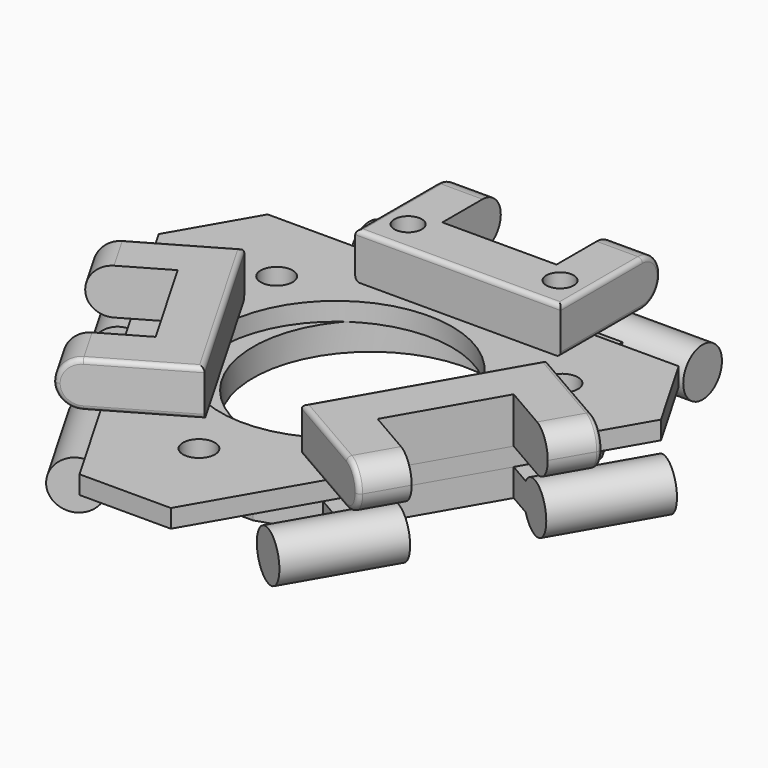
from build123d import *

# Parameters (mm, degrees)
F0_R      = 12.9
F1_DEPTH  = 3
F2_R      = 1.75
F3_DEPTH  = 3.001
F4_R      = 2.65
F5_DEPTH  = 12
F6_R      = 2.65
F7_DEPTH  = 12
F8_R      = 2.65
F9_DEPTH  = 12
F10_R     = 2.65
F11_DEPTH = 12
F12_R     = 2.65
F13_DEPTH = 12
F14_R     = 2.65
F15_DEPTH = 12
F16_R     = 1.75
F16_R_2   = 12.7
F17_DEPTH = 2
F18_SIZE  = 10
F20_DEPTH = 5
F21_R     = 2.49999
F21_2_R   = 2.49999
F21_3_R   = 2.49999
F22_R     = 0.5
F22_2_R   = 0.5
F22_3_R   = 0.5
F23_R     = 1.5
F24_DEPTH = 11.151


# Not quite as in the source:
# - a fillet or chamfer is up to 0.001 mm smaller than in the source, because OpenCascade refuses the exact size


with BuildPart() as f1:
    # F0 (on Top) → F1 (new body)
    with BuildSketch(Plane.XY):
        Polygon((16.0075136901, 22.7174561645), (11.25, 26.956246243), (11.25, 31.956246243), (6.25, 31.956246243), (6.25, 26.956246243), (-6.25, 26.956246243), (-6.25, 31.956246243), (-11.25, 31.956246243), (-11.25, 26.956246243), (-16.0075136901, 22.7174561645), (-19.6075136901, 16.4820732572), (-20.8996567344, 10.2425505034), (-25.2297837534, 7.7425505034), (-22.7297837534, 3.4124234845), (-18.3996567344, 5.9124234845), (-12.1496567344, -4.9128940628), (-16.4797837534, -7.4128940628), (-13.9797837534, -11.7430210817), (-9.6496567344, -9.2430210817), (-3.6, -11.243753757), (3.6, -11.243753757), (9.6497229346, -9.2429064231), (13.9797837534, -11.7430210817), (16.4797837534, -7.4128940628), (12.1496567344, -4.9128940628), (18.3996567344, 5.9124234845), (22.7297837534, 3.4124234845), (25.2297837534, 7.7425505034), (20.8996567344, 10.2425505034), (19.6075136901, 16.4820732572), align=None)
        with Locations((0, 9.3591320669)):
            Circle(F0_R, mode=Mode.SUBTRACT)
    extrude(amount=F1_DEPTH)

    # F2 (on face) → F3 (cut, through all)
    with BuildSketch(Plane.XY.offset(3)):
        with Locations((-14.343412075, 17.5997647108)):
            Circle(F2_R)
        with Locations((14.343412075, 17.5997647108)):
            Circle(F2_R)
        with Locations((0, -7.243753757)):
            Circle(F2_R)
    extrude(amount=-F3_DEPTH, mode=Mode.SUBTRACT)

    # F4 (on face) → F5 (join)
    with BuildSketch(Plane(origin=(6.25, 0, 0), x_dir=(0, -1, 0), z_dir=(-1, 0, 0))):
        with Locations((-31.956246243, 1.5)):
            Circle(F4_R)
    extrude(amount=-F5_DEPTH)

    # F6 (on face) → F7 (join)
    with BuildSketch(Plane.YZ.offset(-6.25)):
        with Locations((31.956246243, 1.5)):
            Circle(F6_R)
    extrude(amount=-F7_DEPTH)

    # F8 (on face) → F9 (join)
    with BuildSketch(Plane(origin=(-7.1600686514, 12.4016026898, 0), x_dir=(0.8660254038, 0.5, 0), z_dir=(0.5, -0.8660254038, 0))):
        with Locations((-17.9783584107, 1.5)):
            Circle(F8_R)
    extrude(amount=-F9_DEPTH)

    # F10 (on face) → F11 (join)
    with BuildSketch(Plane(origin=(-0.9100686514, 1.5762851425, 0), x_dir=(-0.8660254038, -0.5, 0), z_dir=(-0.5, 0.8660254038, 0))):
        with Locations((17.9783584107, 1.5)):
            Circle(F10_R)
    extrude(amount=-F11_DEPTH)

    # F12 (on face) → F13 (join)
    with BuildSketch(Plane(origin=(0.9100686514, 1.5762851425, 0), x_dir=(-0.8660254038, 0.5, 0), z_dir=(0.5, 0.8660254038, 0))):
        with Locations((-17.9783584107, 1.5)):
            Circle(F12_R)
    extrude(amount=-F13_DEPTH)

    # F14 (on face) → F15 (join)
    with BuildSketch(Plane(origin=(7.1600686514, 12.4016026898, 0), x_dir=(0.8660254038, -0.5, 0), z_dir=(-0.5, -0.8660254038, 0))):
        with Locations((17.9783584107, 1.5)):
            Circle(F14_R)
    extrude(amount=-F15_DEPTH)


with BuildPart() as f17:
    # F16 (on face) → F17 (new body)
    with BuildSketch(Plane.XY.offset(3)):
        Polygon((30.1611998525, 26.2840137404), (-34.8388001475, 26.2840137404), (-2.3388001475, -30.0076375056), align=None)
        with Locations((-2.3388001475, -11.243753757)):
            Circle(F16_R, mode=Mode.SUBTRACT)
        with Locations((-17.0792773774, 17.814341432)):
            Circle(F16_R, mode=Mode.SUBTRACT)
        with Locations((-2.3388001475, 7.5201299917)):
            Circle(F16_R_2, mode=Mode.SUBTRACT)
        with Locations((14.343412075, 17.5997647108)):
            Circle(F16_R, mode=Mode.SUBTRACT)
    extrude(amount=F17_DEPTH)

    # F18
    f18_edges = [f17.edges().sort_by_distance(p)[0] for p in [
        (-2.3388, -30.007638, 4),
        (30.1612, 26.284014, 4),
        (-34.8388, 26.284014, 4),
    ]]
    chamfer(f18_edges, length=F18_SIZE)


with BuildPart() as f20:
    # F19 (on face) → F20 (new body)
    with BuildSketch(Plane.XY.offset(5)):
        Polygon((-25.3278599647, 1.9124234845), (-18.3996567344, 5.9124234845), (-12.1496567344, -4.9128940628), (-19.0778599647, -8.9128940628), (-16.5778599647, -13.2430210817), (-5.3195297155, -6.7430210817), (-16.5695297155, 12.7425505034), (-27.8278599647, 6.2425505034), align=None)
    extrude(amount=F20_DEPTH)

    # F21 (radius 2.5 in the source; OpenCascade refuses exactly that, so slightly less here)
    f21_edges = [f20.edges().sort_by_distance(p)[0] for p in [
        (-17.82786, -11.077958, 10),
        (-17.82786, -11.077958, 5),
        (-26.57786, 4.077487, 10),
        (-26.57786, 4.077487, 5),
    ]]
    fillet(f21_edges, radius=F21_R)

    # F22#3
    f22_3_edges = [f20.edges().sort_by_distance(p)[0] for p in [
        (-10.94453, 2.999765, 10),
        (-21.116167, 10.117548, 10),
        (-9.866167, -9.368024, 10),
    ]]
    fillet(f22_3_edges, radius=F22_3_R)


with BuildPart() as f20b:
    # F19 (on face) → F20, piece 2 (new body)
    with BuildSketch(Plane.XY.offset(5)):
        Polygon((19.0901664984, -8.9199992433), (12.1619632681, -4.9199992433), (18.3996567344, 5.9124234845), (25.3278599647, 1.9124234845), (27.8278599647, 6.2425505034), (16.5617732915, 12.7290859796), (5.3350718844, -6.7699195482), (16.5901664984, -13.2501262623), align=None)
    extrude(amount=F20_DEPTH)

    # F21#2 (radius 2.5 in the source; OpenCascade refuses exactly that, so slightly less here)
    f21_2_edges = [f20b.edges().sort_by_distance(p)[0] for p in [
        (17.840166, -11.085063, 10),
        (17.840166, -11.085063, 5),
        (26.57786, 4.077487, 10),
        (26.57786, 4.077487, 5),
    ]]
    fillet(f21_2_edges, radius=F21_2_R)

    # F22#2
    f22_2_edges = [f20b.edges().sort_by_distance(p)[0] for p in [
        (10.948423, 2.979583, 10),
        (9.879345, -9.386319, 10),
        (21.111542, 10.109522, 10),
    ]]
    fillet(f22_2_edges, radius=F22_2_R)


with BuildPart() as f20c:
    # F19 (on face) → F20, piece 3 (new body)
    with BuildSketch(Plane.XY.offset(5)):
        Polygon((11.25, 34.956246243), (6.25, 34.956246243), (6.25, 26.956246243), (-6.25, 26.956246243), (-6.25, 34.956246243), (-11.25, 34.956246243), (-11.25, 21.2840137404), (11.25, 21.2840137404), align=None)
    extrude(amount=F20_DEPTH)

    # F21#3 (radius 2.5 in the source; OpenCascade refuses exactly that, so slightly less here)
    f21_3_edges = [f20c.edges().sort_by_distance(p)[0] for p in [
        (-8.75, 34.956246, 10),
        (-8.75, 34.956246, 5),
        (8.75, 34.956246, 5),
        (8.75, 34.956246, 10),
    ]]
    fillet(f21_3_edges, radius=F21_3_R)

    # F22
    f22_edges = [f20c.edges().sort_by_distance(p)[0] for p in [
        (0, 21.284014, 10),
        (11.25, 26.870135, 10),
        (-11.25, 26.870135, 10),
    ]]
    fillet(f22_edges, radius=F22_R)


with BuildPart() as f24_tool:
    # F23 (on face) → F24 (new body, through all)
    with BuildSketch(Plane.XY.offset(10)):
        with Locations((-8.3209636769, 24.8603269392)):
            Circle(F23_R)
        with Locations((8.3209636769, 24.8603269392)):
            Circle(F23_R)
    extrude(amount=-F24_DEPTH)


with BuildPart() as f17_1:
    add(f17.part)

    # F24: cut by f24_tool
    add(f24_tool.part, mode=Mode.SUBTRACT)


with BuildPart() as f20c_1:
    add(f20c.part)

    # F24: cut by f24_tool
    add(f24_tool.part, mode=Mode.SUBTRACT)


solid = Compound([f1.part, f20.part, f20b.part, f17_1.part, f20c_1.part])
